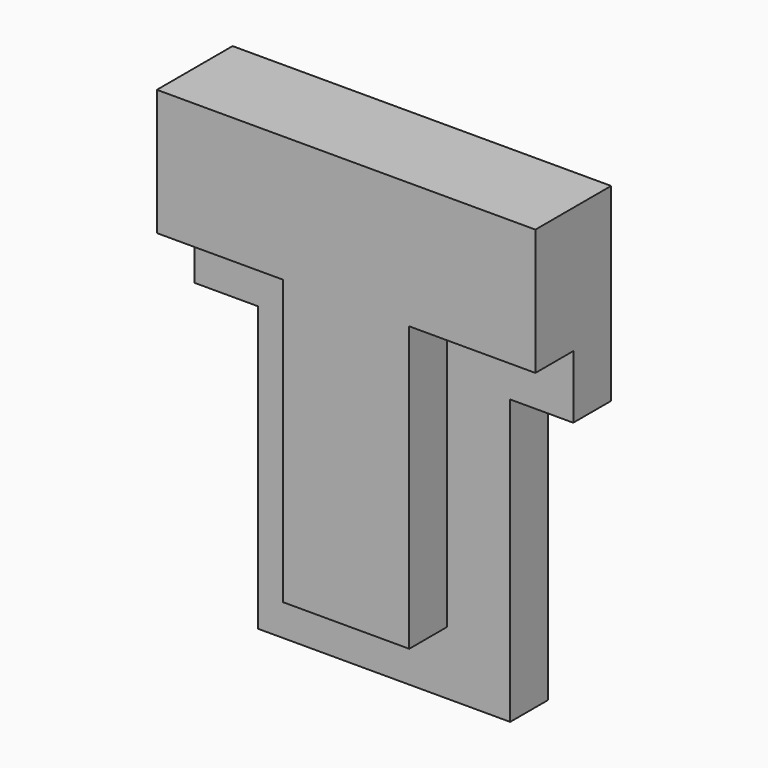
from build123d import *

# Parameters (mm, degrees)
F1_DEPTH = 7.62
F2_DEPTH = 3.81


# Not quite as in the source:
# - a feature names something its author has since deleted; it is built from what else it names


with BuildPart() as f1:
    # F0 (on Front) → F1 (new body)
    with BuildSketch(Plane.XZ):
        Polygon((-20.32, 5.08), (-20.32, -17.78), (-10.16, -17.78), (-10.16, 5.08), (0, 5.08), (0, 15.24), (-30.48, 15.24), (-30.48, 5.08), align=None)
    extrude(amount=F1_DEPTH)

    # F0 (on Front) → F2 (join)
    with BuildSketch(Plane.XZ):
        Polygon((-10.16, 5.08), (-10.16, -17.78), (-5.08, -17.78), (-5.08, 0), (0, 0), (0, 5.08), align=None)
        Polygon((-20.32, -17.78), (-25.4, -17.78), (-25.4, -22.86), (-5.08, -22.86), (-5.08, -17.78), (-10.16, -17.78), align=None)
        Polygon((-25.4, 0), (-25.4, -17.78), (-20.32, -17.78), (-20.32, 5.08), (-30.48, 5.08), (-30.48, 0), align=None)
    extrude(amount=F2_DEPTH)


solid = f1.part
